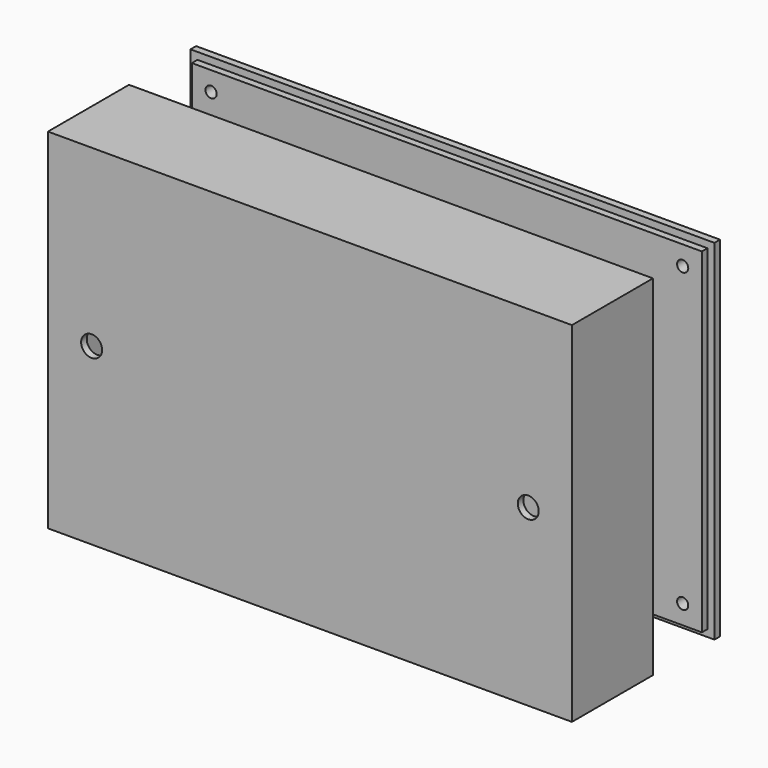
from build123d import *

# Parameters (mm, degrees)
F0_W     = 81.5
F0_H     = 23.5
F0_W_2   = 79
F0_H_2   = 21
F1_DEPTH = 5
F0_W_3   = 150
F0_H_3   = 100
F0_W_4   = 146
F0_H_4   = 96
F0_R     = 3.5
F0_R_2   = 3
F0_R_3   = 1.5
F2_DEPTH = 2
F3_DEPTH = 27
F5_W     = 150
F5_H     = 100
F5_W_2   = 146
F5_H_2   = 96
F5_R     = 1.6
F6_DEPTH = 2
F7_DEPTH = 2


# Not quite as in the source:
# - a feature of the source that left no trace in its solid (it failed there, or was rolled back) is left out


with BuildPart() as f1:
    # F0 (on Front) → F1 (new body)
    with BuildSketch(Plane.XZ):
        with Locations((61.7559325695, 122.2460778952)):
            Rectangle(F0_W, F0_H)
        with Locations((61.7559325695, 122.2460778952)):
            Rectangle(F0_W_2, F0_H_2, mode=Mode.SUBTRACT)
    extrude(amount=-F1_DEPTH)


with BuildPart() as f2:
    # F0 (on Front) → F2 (new body)
    with BuildSketch(Plane.XZ):
        with Locations((61.7559325695, 122.2460778952)):
            Rectangle(F0_W_3, F0_H_3)
        with Locations((61.7559325695, 122.2460778952)):
            Rectangle(F0_W_4, F0_H_4, mode=Mode.SUBTRACT)
        with Locations((61.7559325695, 122.2460778952)):
            Rectangle(F0_W_4, F0_H_4)
        with Locations((-5.7440674305, 79.7460778952)):
            Circle(F0_R, mode=Mode.SUBTRACT)
        with Locations((61.7559325695, 122.2460778952)):
            Rectangle(F0_W, F0_H, mode=Mode.SUBTRACT)
        with Locations((129.2559325695, 79.7460778952)):
            Circle(F0_R, mode=Mode.SUBTRACT)
        with Locations((-0.7440674305, 122.2460778952)):
            Circle(F0_R_2, mode=Mode.SUBTRACT)
        with Locations((-5.7440674305, 164.7460778952)):
            Circle(F0_R, mode=Mode.SUBTRACT)
        with Locations((124.2559325695, 122.2460778952)):
            Circle(F0_R_2, mode=Mode.SUBTRACT)
        with Locations((129.2559325695, 164.7460778952)):
            Circle(F0_R, mode=Mode.SUBTRACT)
        with Locations((61.7559325695, 122.2460778952)):
            Rectangle(F0_W, F0_H)
        with Locations((61.7559325695, 122.2460778952)):
            Rectangle(F0_W_2, F0_H_2, mode=Mode.SUBTRACT)
        with Locations((61.7559325695, 122.2460778952)):
            Rectangle(F0_W_2, F0_H_2)
        with Locations((-5.7440674305, 79.7460778952)):
            Circle(F0_R)
        with Locations((-5.7440674305, 79.7460778952)):
            Circle(F0_R_3, mode=Mode.SUBTRACT)
        with Locations((129.2559325695, 164.7460778952)):
            Circle(F0_R)
        with Locations((129.2559325695, 164.7460778952)):
            Circle(F0_R_3, mode=Mode.SUBTRACT)
        with Locations((129.2559325695, 79.7460778952)):
            Circle(F0_R)
        with Locations((129.2559325695, 79.7460778952)):
            Circle(F0_R_3, mode=Mode.SUBTRACT)
        with Locations((-5.7440674305, 164.7460778952)):
            Circle(F0_R)
        with Locations((-5.7440674305, 164.7460778952)):
            Circle(F0_R_3, mode=Mode.SUBTRACT)
        with Locations((-5.7440674305, 79.7460778952)):
            Circle(F0_R_3)
        with Locations((129.2559325695, 164.7460778952)):
            Circle(F0_R_3)
        with Locations((129.2559325695, 79.7460778952)):
            Circle(F0_R_3)
        with Locations((-5.7440674305, 164.7460778952)):
            Circle(F0_R_3)
    extrude(amount=F2_DEPTH)

    # F0 (on Front) → F3 (join)
    with BuildSketch(Plane.XZ):
        with Locations((61.7559325695, 122.2460778952)):
            Rectangle(F0_W_3, F0_H_3)
        with Locations((61.7559325695, 122.2460778952)):
            Rectangle(F0_W_4, F0_H_4, mode=Mode.SUBTRACT)
        with Locations((129.2559325695, 164.7460778952)):
            Circle(F0_R)
        with Locations((129.2559325695, 164.7460778952)):
            Circle(F0_R_3, mode=Mode.SUBTRACT)
        with Locations((-5.7440674305, 164.7460778952)):
            Circle(F0_R)
        with Locations((-5.7440674305, 164.7460778952)):
            Circle(F0_R_3, mode=Mode.SUBTRACT)
        with Locations((-5.7440674305, 79.7460778952)):
            Circle(F0_R)
        with Locations((-5.7440674305, 79.7460778952)):
            Circle(F0_R_3, mode=Mode.SUBTRACT)
        with Locations((129.2559325695, 79.7460778952)):
            Circle(F0_R)
        with Locations((129.2559325695, 79.7460778952)):
            Circle(F0_R_3, mode=Mode.SUBTRACT)
    extrude(amount=-F3_DEPTH)


with BuildPart() as f6:
    # F5 (on offset) → F6 (new body)
    with BuildSketch(Plane.XZ.offset(-49)):
        with Locations((61.7559325695, 122.2460778952)):
            Rectangle(F5_W, F5_H)
        with Locations((61.7559325695, 122.2460778952)):
            Rectangle(F5_W_2, F5_H_2, mode=Mode.SUBTRACT)
        with Locations((61.7559325695, 122.2460778952)):
            Rectangle(F5_W_2, F5_H_2)
        with Locations((-5.7440674305, 79.7460778952)):
            Circle(F5_R, mode=Mode.SUBTRACT)
        with Locations((129.2559325695, 79.7460778952)):
            Circle(F5_R, mode=Mode.SUBTRACT)
        with Locations((-5.7440674305, 164.7460778952)):
            Circle(F5_R, mode=Mode.SUBTRACT)
        with Locations((129.2559325695, 164.7460778952)):
            Circle(F5_R, mode=Mode.SUBTRACT)
    extrude(amount=-F6_DEPTH)

    # F5 (on offset) → F7 (join)
    with BuildSketch(Plane.XZ.offset(-49)):
        with Locations((61.7559325695, 122.2460778952)):
            Rectangle(F5_W_2, F5_H_2)
        with Locations((-5.7440674305, 79.7460778952)):
            Circle(F5_R, mode=Mode.SUBTRACT)
        with Locations((129.2559325695, 79.7460778952)):
            Circle(F5_R, mode=Mode.SUBTRACT)
        with Locations((-5.7440674305, 164.7460778952)):
            Circle(F5_R, mode=Mode.SUBTRACT)
        with Locations((129.2559325695, 164.7460778952)):
            Circle(F5_R, mode=Mode.SUBTRACT)
    extrude(amount=F7_DEPTH)


solid = Compound([f1.part, f2.part, f6.part])
